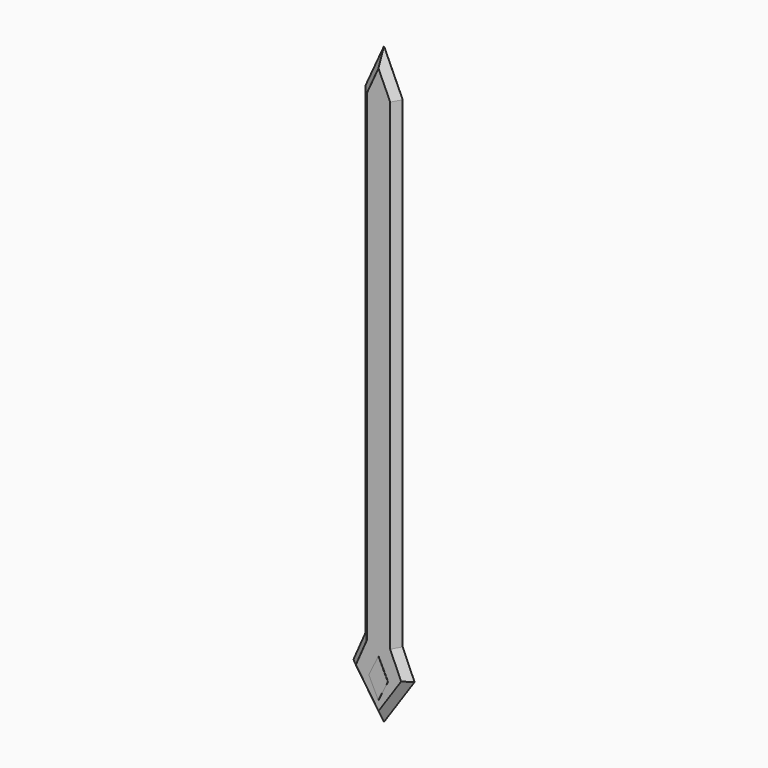
from build123d import *

# Parameters (mm, degrees)
F1_DEPTH = 6.35
F2_DEPTH = 6.35
F3_SIZE2 = 6.34999
F3_SIZE  = 6.34999
F4_DEPTH = 0.127
F5_DEPTH = 0.127
F7_DEPTH = 0.254
F8_DEPTH = 12.954


# Not quite as in the source:
# - a fillet or chamfer is up to 0.001 mm smaller than in the source, because OpenCascade refuses the exact size


with BuildPart() as f1:
    # F0 (on Front) → F1 (new body)
    with BuildSketch(Plane.XZ):
        Polygon((-17.139416188, 28.1973872334), (-27.9807504267, 3.4191238228), (0, -37.7674587071), (27.964355424, 3.4191238228), (17.08493568, 28.1973872334), (17.08493568, 469.1244959831), (0, 506.7884922028), (-17.139416188, 469.1244959831), align=None)
    extrude(amount=F1_DEPTH)

    # F2 (add): a face of the model
    f2_faces = [f1.faces().sort_by_distance(p)[0] for p in [
        (-0.0248835797, 0, 225.9211420486),
    ]]
    extrude(f2_faces, amount=F2_DEPTH)

    # F3 (size 6.35 and 6.35 in the source; OpenCascade refuses exactly that, so slightly less here)
    f3_edges = [f1.edges().sort_by_distance(p)[0] for p in [
        (-22.560083, -6.35, 15.808256),
        (-13.990375, -6.35, -17.174167),
        (13.982178, -6.35, -17.174167),
        (22.524646, -6.35, 15.808256),
        (17.084936, -6.35, 248.660942),
        (8.542468, -6.35, 487.956494),
        (-8.569708, -6.35, 487.956494),
        (-17.139416, -6.35, 248.660942),
        (-22.560083, 6.35, 15.808256),
        (-13.990375, 6.35, -17.174167),
        (13.982178, 6.35, -17.174167),
        (22.524646, 6.35, 15.808256),
        (17.084936, 6.35, 248.660942),
        (8.542468, 6.35, 487.956494),
        (-8.569708, 6.35, 487.956494),
        (-17.139416, 6.35, 248.660942),
    ]]
    chamfer(f3_edges, length=F3_SIZE, length2=F3_SIZE2)

    # F4 (cut): a face of the model
    f4_faces = [f1.faces().sort_by_distance(p)[0] for p in [
        (-0.0252861091, -6.35, 223.0026633937),
    ]]
    extrude(f4_faces, amount=-F4_DEPTH, mode=Mode.SUBTRACT)

    # F5 (cut): a face of the model
    f5_faces = [f1.faces().sort_by_distance(p)[0] for p in [
        (-0.0252861091, 6.35, 223.0026633937),
    ]]
    extrude(f5_faces, amount=-F5_DEPTH, mode=Mode.SUBTRACT)

    # F6 (on face) → F7 (join)
    with BuildSketch(Plane.XZ.offset(6.223)):
        Polygon((8.6913099512, 0), (0, 17.8065411747), (-8.6860535666, 0), (0, -17.7944861352), align=None)
    extrude(amount=F7_DEPTH)

    # F8 (add): a face of the model
    f8_faces = [f1.faces().sort_by_distance(p)[0] for p in [
        (0.0017521282, -6.477, 0.0040183465),
    ]]
    extrude(f8_faces, amount=-F8_DEPTH)


solid = f1.part
